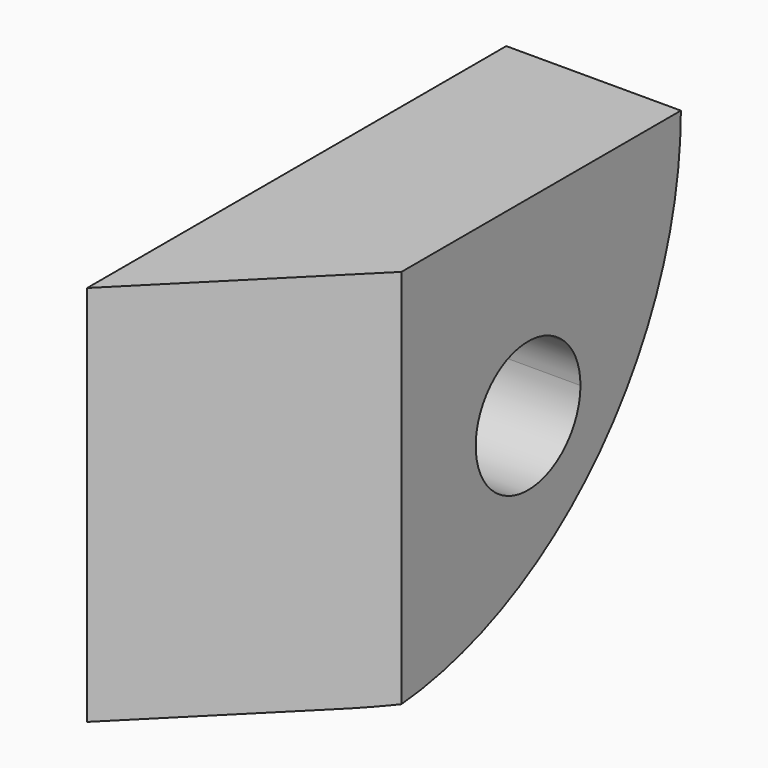
from build123d import *

# Parameters (mm, degrees)
F0_W     = 76.2
F0_H     = 55.5625
F1_DEPTH = 25.4
F2_R     = 55.56249
F4_DEPTH = 25.4
F6_DEPTH = 55.5635


# Not quite as in the source:
# - a fillet or chamfer is up to 0.001 mm smaller than in the source, because OpenCascade refuses the exact size


with BuildPart() as f1:
    # F0 (on Right) → F1 (new body)
    with BuildSketch(Plane.YZ):
        Rectangle(F0_W, F0_H)
    extrude(amount=F1_DEPTH)

    # F2 (radius 55.5625 in the source; OpenCascade refuses exactly that, so slightly less here)
    f2_edges = [f1.edges().sort_by_distance(p)[0] for p in [
        (12.7, 38.1, -27.78125),
    ]]
    fillet(f2_edges, radius=F2_R)

    # F3 (on face) → F4 (cut)
    with BuildSketch(Plane.YZ.offset(25.4)):
        with BuildLine():
            ThreePointArc((17.0539420908, 6.7351920908), (3.5835579092, 6.7351920908), (3.5835579092, -6.7351920908))
            Line((3.5835579092, -6.7351920908), (17.0539420908, 6.7351920908))
        make_face()
        with BuildLine():
            Line((17.0539420908, 6.7351920908), (3.5835579092, -6.7351920908))
            ThreePointArc((3.5835579092, -6.7351920908), (13.9638096933, -8.7999525472), (19.84375, 0))
            ThreePointArc((19.84375, 0), (19.1187025472, 3.6450596933), (17.0539420908, 6.7351920908))
        make_face()
    extrude(amount=-F4_DEPTH, mode=Mode.SUBTRACT)

    # F5 (on face) → F6 (cut, through all)
    with BuildSketch(Plane.XY.offset(27.78125)):
        Polygon((25.4, -12.7), (0, -38.1), (25.4, -38.1), align=None)
    extrude(amount=-F6_DEPTH, mode=Mode.SUBTRACT)


solid = f1.part
